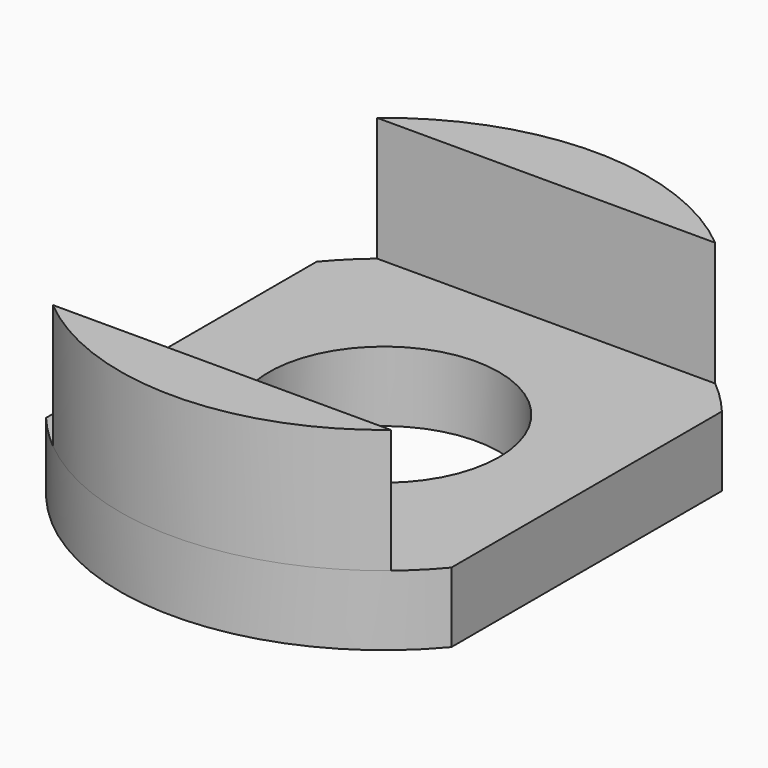
from build123d import *

# Parameters (mm, degrees)
F0_R     = 19.6
F0_R_2   = 8.55
F1_DEPTH = 5.2
F3_DEPTH = 9.2
F4_DEPTH = 5.201


with BuildPart() as f1:
    # F0 (on Top) → F1 (new body)
    with BuildSketch(Plane.XY):
        Circle(F0_R)
        Circle(F0_R_2, mode=Mode.SUBTRACT)
    extrude(amount=F1_DEPTH)

    # F2 (on face) → F3 (join)
    with BuildSketch(Plane.XY.offset(5.2)):
        with BuildLine():
            ThreePointArc((-12.5561737803, -15.05), (0, -19.6), (12.5561737803, -15.05))
            Line((12.5561737803, -15.05), (-12.5561737803, -15.05))
        make_face()
        with BuildLine():
            Line((-12.5561737803, 15.05), (12.5561737803, 15.05))
            ThreePointArc((12.5561737803, 15.05), (0, 19.6), (-12.5561737803, 15.05))
        make_face()
    extrude(amount=F3_DEPTH)

    # F2 (on face) → F4 (cut, through all)
    with BuildSketch(Plane.XY.offset(5.2)):
        with BuildLine():
            ThreePointArc((-15.05, 12.5561737803), (-19.6, 0), (-15.05, -12.5561737803))
            Line((-15.05, -12.5561737803), (-15.05, 12.5561737803))
        make_face()
        with BuildLine():
            Line((15.05, 12.5561737803), (15.05, -12.5561737803))
            ThreePointArc((15.05, -12.5561737803), (18.4274252135, -6.6775744099), (19.6, 0))
            ThreePointArc((19.6, 0), (18.4274252135, 6.6775744099), (15.05, 12.5561737803))
        make_face()
    extrude(amount=-F4_DEPTH, mode=Mode.SUBTRACT)


solid = f1.part
